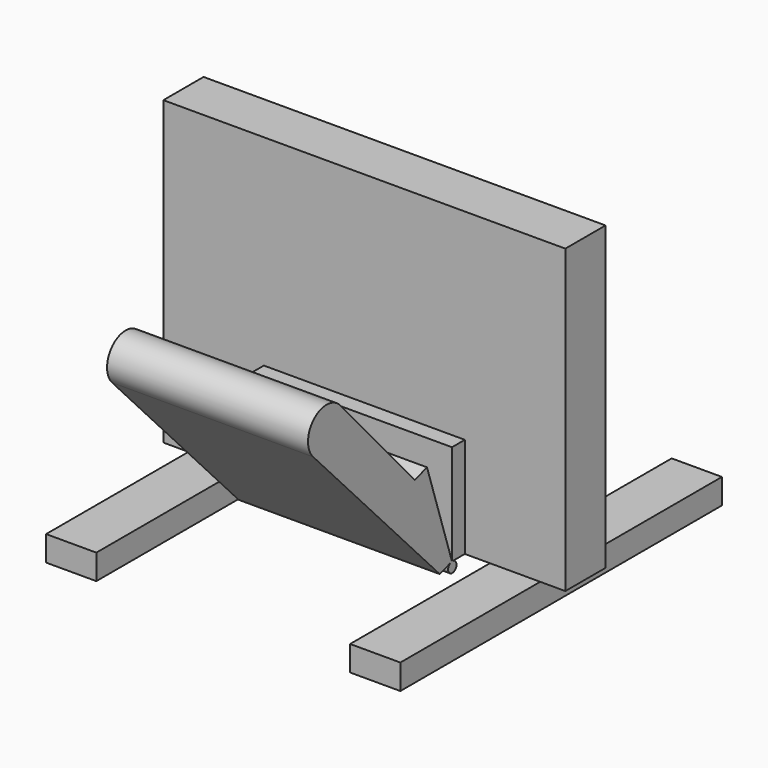
from build123d import *

# Parameters (mm, degrees)
F0_W      = 101.6
F0_H      = 76.2
F1_DEPTH  = 12.7
F2_W      = 50.8
F2_H      = 25.4
F3_DEPTH  = 4.064
F5_DEPTH  = 50.8
F7_DEPTH  = 50.8
F9_DEPTH  = 50.8
F10_W     = 12.7
F10_H     = 101.6
F11_DEPTH = 6.35
F12_W     = 12.7
F12_H     = 101.6
F13_DEPTH = 6.35


with BuildPart() as f1:
    # F0 (on Front) → F1 (new body)
    with BuildSketch(Plane.XZ):
        with Locations((50.8, 38.1)):
            Rectangle(F0_W, F0_H)
    extrude(amount=F1_DEPTH)

    # F2 (on face) → F3 (join)
    with BuildSketch(Plane.XZ.offset(12.7)):
        with Locations((50.8, 12.7)):
            Rectangle(F2_W, F2_H)
    extrude(amount=F3_DEPTH)

    # F4 (on face) → F5 (join)
    with BuildSketch(Plane.YZ.offset(76.2)):
        Polygon((-20.6267049946, -1.2631730384), (-16.764, 0), (-24.6588314903, 24.1419062159), (-28.5215364849, 22.8787331775), align=None)
    extrude(amount=-F5_DEPTH)

    # F6 (on face) → F7 (join)
    with BuildSketch(Plane.YZ.offset(76.2)):
        with BuildLine():
            Line((-16.5507770221, 0), (-16.764, 0))
            ThreePointArc((-16.764, 0), (-17.5513062441, -2.2836680049), (-15.3387688414, -1.31430279))
            ThreePointArc((-15.3387688414, -1.31430279), (-15.6880232962, -0.4203850569), (-16.5507770221, 0))
        make_face()
        with BuildLine():
            ThreePointArc((-16.5507770221, 0), (-16.6573885111, 0.0043168797), (-16.764, 0))
            Line((-16.764, 0), (-16.5507770221, 0))
        make_face()
    extrude(amount=-F7_DEPTH)

    # F8 (on face) → F9 (join)
    with BuildSketch(Plane.YZ.offset(76.2)):
        with BuildLine():
            Line((-20.6267049946, -1.2631730384), (-28.5215364849, 22.8787331775))
            Line((-28.5215364849, 22.8787331775), (-52.1061010659, 49.1076633334))
            ThreePointArc((-52.1061010659, 49.1076633334), (-60.3932888084, 49.3824101727), (-60.6419928372, 41.0943999887))
            Line((-60.6419928372, 41.0943999887), (-20.6267049946, -1.2631730384))
        make_face()
    extrude(amount=-F9_DEPTH)

    # F10 (on face) → F11 (join)
    with BuildSketch(Plane(origin=(0, 0, 0), x_dir=(1, 0, 0), z_dir=(0, 0, -1))):
        with Locations((88.9, 6.0887979344)):
            Rectangle(F10_W, F10_H)
    extrude(amount=F11_DEPTH)

    # F12 (on face) → F13 (join)
    with BuildSketch(Plane(origin=(0, 0, 0), x_dir=(1, 0, 0), z_dir=(0, 0, -1))):
        with Locations((12.7, 6.8910890259)):
            Rectangle(F12_W, F12_H)
    extrude(amount=F13_DEPTH)


solid = f1.part
